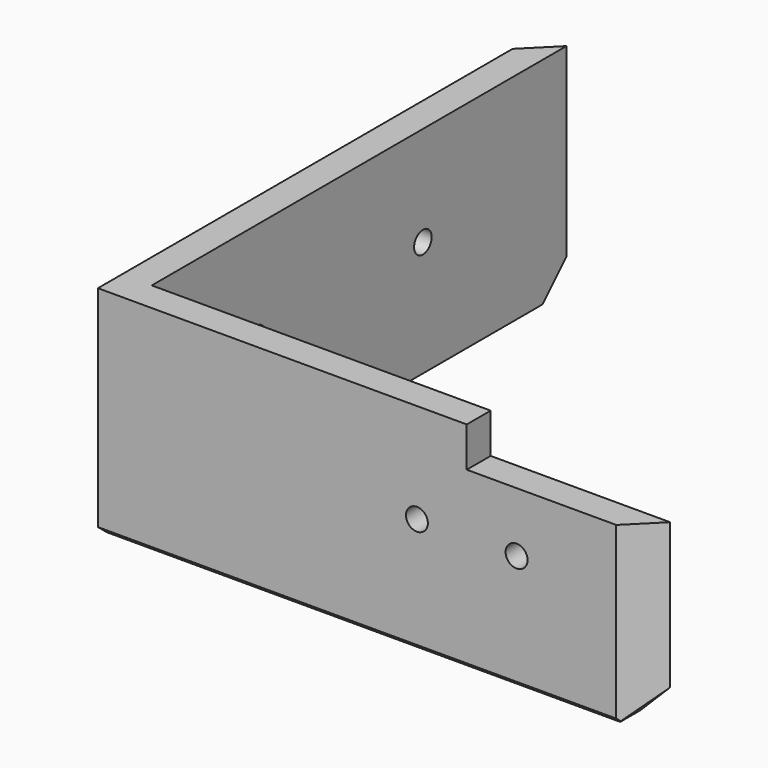
from build123d import *

# Parameters (mm, degrees)
F1_DEPTH  = 21.6
F2_W      = 52
F2_H      = 52
F3_DEPTH  = 22
F4_SIZE   = 2.99999
F5_SIZE   = 0.5
F6_R      = 1.1
F7_DEPTH  = 3
F8_R      = 1.1
F9_DEPTH  = 3
F10_W     = 18
F10_H     = 4
F11_DEPTH = 3


# Not quite as in the source:
# - a fillet or chamfer is up to 0.001 mm smaller than in the source, because OpenCascade refuses the exact size


with BuildPart() as f1:
    # F0 (on Top) → F1 (new body)
    with BuildSketch(Plane.XY):
        Polygon((-12.1071431786, 40.3610856729), (-12.1071431786, -14.6389143271), (42.8928568214, -14.6389143271), (42.8928568214, 7.8610856729), (10.3928568214, 40.3610856729), align=None)
    extrude(amount=F1_DEPTH)

    # F2 (on face) → F3 (cut)
    with BuildSketch(Plane.XY.offset(21.6)):
        with Locations((16.8928568214, 14.3610856729)):
            Rectangle(F2_W, F2_H)
    extrude(amount=-F3_DEPTH, mode=Mode.SUBTRACT)

    # F4 (size 3 in the source; OpenCascade refuses exactly that, so slightly less here)
    f4_edges = [f1.edges().sort_by_distance(p)[0] for p in [
        (42.892857, -13.138914, 0),
        (-10.607143, 40.361086, 0),
        (-12.107143, 40.361086, 10.8),
        (42.892857, -14.638914, 10.8),
    ]]
    chamfer(f4_edges, length=F4_SIZE)

    # F5
    f5_edges = [f1.edges().sort_by_distance(p)[0] for p in [
        (13.892862, -14.638914, 0),
        (-12.107143, 11.361091, 0),
    ]]
    chamfer(f5_edges, length=F5_SIZE)

    # F6 (on face) → F7 (cut)
    with BuildSketch(Plane.XZ.offset(14.6389143271)):
        with Locations((29.8928568214, 11.6)):
            Circle(F6_R)
        with Locations((19.8928568214, 11.6)):
            Circle(F6_R)
    extrude(amount=-F7_DEPTH, mode=Mode.SUBTRACT)

    # F8 (on face) → F9 (cut)
    with BuildSketch(Plane(origin=(-12.1071431786, 0, 0), x_dir=(0, -1, 0), z_dir=(-1, 0, 0))):
        with Locations((-22.3610856729, 11.6)):
            Circle(F8_R)
        with Locations((-1.5111208195, 11.6)):
            Circle(F8_R)
    extrude(amount=-F9_DEPTH, mode=Mode.SUBTRACT)

    # F10 (on face) → F11 (cut)
    with BuildSketch(Plane(origin=(0, -11.6389143271, 0), x_dir=(-1, 0, 0), z_dir=(0, 1, 0))):
        with Locations((-33.8928568214, 19.6)):
            Rectangle(F10_W, F10_H)
    extrude(amount=-F11_DEPTH, mode=Mode.SUBTRACT)


solid = f1.part
